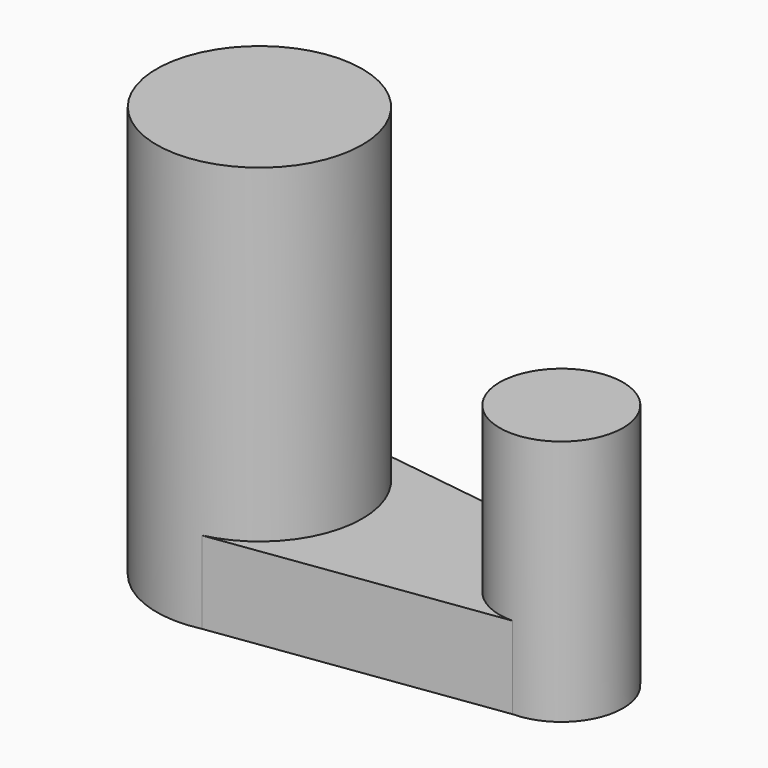
from build123d import *

# Parameters (mm, degrees)
F1_DEPTH = 3
F2_DEPTH = 15
F3_DEPTH = 9


with BuildPart() as f1:
    # F0 (on Top) → F1 (new body)
    with BuildSketch(Plane.XY):
        with BuildLine():
            ThreePointArc((-4.4288796676, -3.6796678124), (-2.3253257096, -2.3633430927), (-1.5043057066, -0.0216394017))
            ThreePointArc((-1.5043057066, -0.0216394017), (-2.3253257096, 2.3200642894), (-4.4288796676, 3.6363890091))
            ThreePointArc((-4.4288796676, 3.6363890091), (-9.0043057066, -0.0216394017), (-4.4288796676, -3.6796678124))
        make_face()
        with BuildLine():
            ThreePointArc((-4.4288796676, 3.6363890091), (-2.3253257096, 2.3200642894), (-1.5043057066, -0.0216394017))
            ThreePointArc((-1.5043057066, -0.0216394017), (-2.3253257096, -2.3633430927), (-4.4288796676, -3.6796678124))
            Line((-4.4288796676, -3.6796678124), (5.7708010962, -2.262551744))
            ThreePointArc((5.7708010962, -2.262551744), (3.4956906544, -0.0126918671), (5.7708010962, 2.2371680098))
            Line((5.7708010962, 2.2371680098), (-4.4288796676, 3.6363890091))
        make_face()
        with BuildLine():
            ThreePointArc((7.9956906544, -0.0126918671), (7.3455341614, 1.5693955998), (5.7708010962, 2.2371680098))
            ThreePointArc((5.7708010962, 2.2371680098), (3.4956906544, -0.0126918671), (5.7708010962, -2.262551744))
            ThreePointArc((5.7708010962, -2.262551744), (7.3455341614, -1.594779334), (7.9956906544, -0.0126918671))
        make_face()
    extrude(amount=F1_DEPTH)

    # F0 (on Top) → F2 (join)
    with BuildSketch(Plane.XY):
        with BuildLine():
            ThreePointArc((-4.4288796676, -3.6796678124), (-2.3253257096, -2.3633430927), (-1.5043057066, -0.0216394017))
            ThreePointArc((-1.5043057066, -0.0216394017), (-2.3253257096, 2.3200642894), (-4.4288796676, 3.6363890091))
            ThreePointArc((-4.4288796676, 3.6363890091), (-9.0043057066, -0.0216394017), (-4.4288796676, -3.6796678124))
        make_face()
    extrude(amount=F2_DEPTH)

    # F0 (on Top) → F3 (join)
    with BuildSketch(Plane.XY):
        with BuildLine():
            ThreePointArc((7.9956906544, -0.0126918671), (7.3455341614, 1.5693955998), (5.7708010962, 2.2371680098))
            ThreePointArc((5.7708010962, 2.2371680098), (3.4956906544, -0.0126918671), (5.7708010962, -2.262551744))
            ThreePointArc((5.7708010962, -2.262551744), (7.3455341614, -1.594779334), (7.9956906544, -0.0126918671))
        make_face()
    extrude(amount=F3_DEPTH)


solid = f1.part
